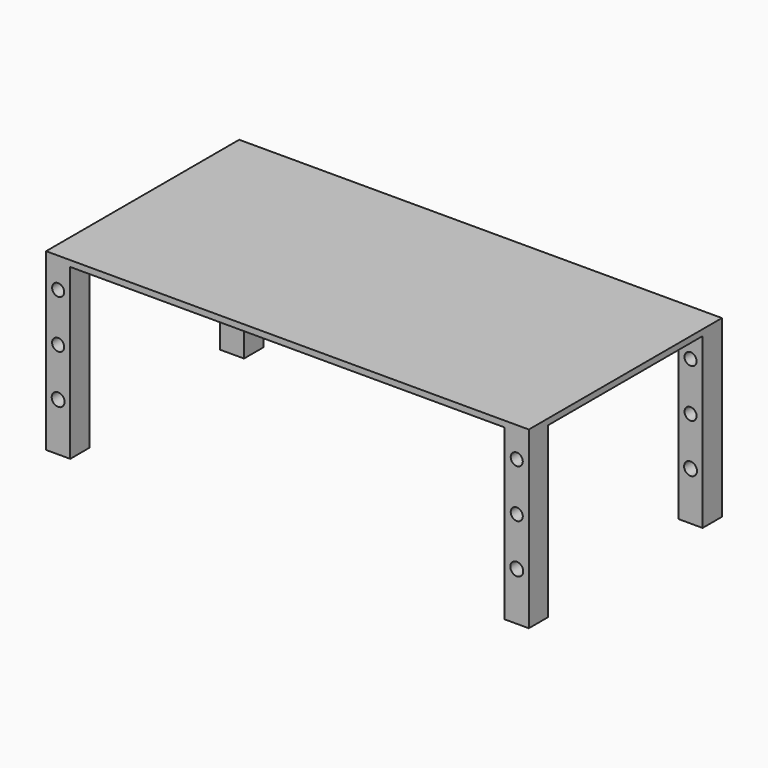
from build123d import *

# Parameters (mm, degrees)
F0_W     = 2000
F0_H     = 1000
F1_DEPTH = 25
F2_W     = 100
F2_H     = 100
F4_DEPTH = 700
F3_R     = 25
F3_R_2   = 26.6431742527
F5_DEPTH = 1000.001
F6_R     = 138.4561690077
F7_W     = 118.5409426689
F7_H     = 157.5430333614
F9_T     = 2.5


# Not quite as in the source:
# - a pattern or mirror of a feature is missing from the dataset's text; its kind, count and spacing are read off the source's solid
# - a shell that OpenCascade refuses in one call is made with other operations: the cavity is built on its own and cut out


with BuildPart() as f1:
    # F0 (on Top) → F1 (new body)
    with BuildSketch(Plane.XY):
        Rectangle(F0_W, F0_H)
    extrude(amount=F1_DEPTH)

    # F2 (on face) → F4 (join)
    with BuildSketch(Plane(origin=(0, 0, 0), x_dir=(1, 0, 0), z_dir=(0, 0, -1))):
        with Locations((-950, 450)):
            Rectangle(F2_W, F2_H)
        with Locations((-950, -450)):
            Rectangle(F2_W, F2_H)
    f4 = extrude(amount=F4_DEPTH)

    # F4_copies: F4 across plane
    add(f4.mirror(Plane(origin=(0, 0, 0), x_dir=(0, 0, 1), z_dir=(1, 0, 0))))

    # F3 (on face) → F5 (cut, through all)
    with BuildSketch(Plane.XZ.offset(500)):
        with Locations((-950, -100)):
            Circle(F3_R)
        with Locations((-950, -300)):
            Circle(F3_R)
        with Locations((-950, -500)):
            Circle(F3_R_2)
    f5 = extrude(amount=-F5_DEPTH, mode=Mode.SUBTRACT)

    # F5_copies: F5 across plane
    add(f5.mirror(Plane(origin=(0, 0, 0), x_dir=(0, 0, 1), z_dir=(1, 0, 0))), mode=Mode.SUBTRACT)


with BuildPart() as f8:
    # F6 (on face) → F8 section 0
    with BuildSketch(Plane.XZ.offset(500)):
        with Locations((508.7250471115, -680.1778674126)):
            Circle(F6_R)
    # F7 (on face) → F8 section 1
    with BuildSketch(Plane.YZ.offset(-900)):
        with Locations((720.3351557255, -315.4024332762)):
            Rectangle(F7_W, F7_H)
    loft()

    # F9: shell of thickness 2.5, made by hand


with BuildPart() as f9_core1:
    # F9_t2: copy of F8
    add(f8.part)

    # the walls: a layer under each face that stays
    f9_faces = [f9_core1.faces().sort_by_distance(p)[0] for p in [
        (508.7250471115, -500, -680.1778674126),
        (-900, 720.3351557255, -315.4024332762),
    ]]
    thicken(f9_faces, amount=-F9_T, mode=Mode.SUBTRACT)


with BuildPart() as f8_1:
    add(f8.part)

    # what is left inside the walls is the cavity
    f9_cavity = [f9_core1.part.solids().sort_by_distance(p)[0] for p in [
        (-53.137215, -112.959985, -558.586056),
    ]]
    add(f9_cavity, mode=Mode.SUBTRACT)


solid = f1.part
